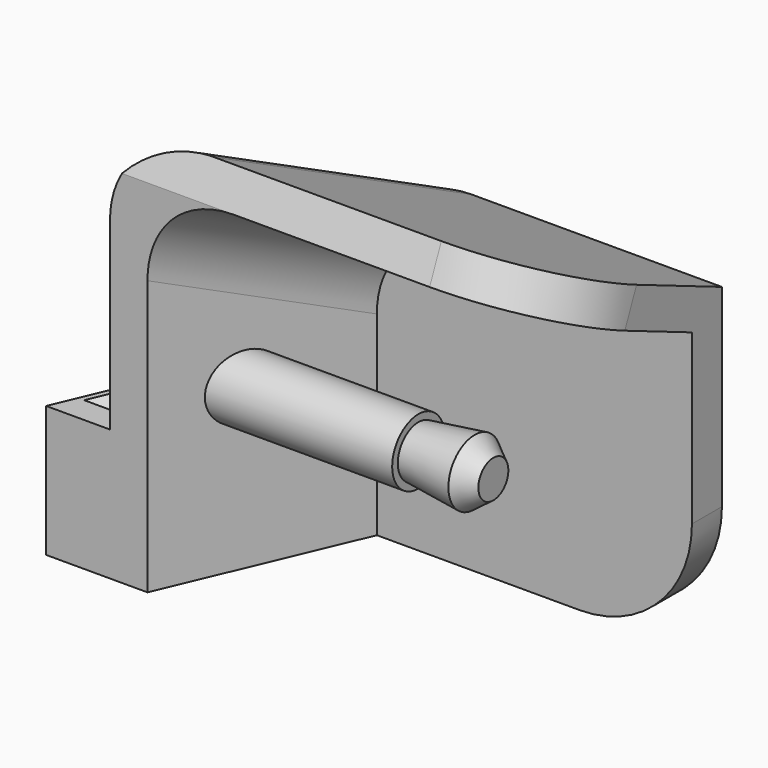
from build123d import *

# Parameters (mm, degrees)
F4_DEPTH      = 20
F4_DEPTH_BACK = 5
F6_DEPTH      = 2
F8_DEPTH      = 2
F10_DEPTH     = 25
F11_REACH     = 32.8764516567
F14_REACH     = 25.371169227
F16_DEPTH     = 7
F17_SIZE      = 1
F18_T4_DEPTH  = 33.0979417074
F18_T8_DEPTH  = 34.519175586


# Not quite as in the source:
# - a fillet or chamfer that OpenCascade refuses, or shapes differently, is made with other operations: its cross-section is extruded or revolved along the edge and cut away or added
# - a feature names something its author has since deleted; it is built from what else it names


with BuildPart() as f1:
    # F0 (on Front) → F1 (revolve)
    with BuildSketch(Plane.XZ):
        Polygon((-4, 1.75), (-14, 1.75), (-14, 0), (0, 0), (0, 1), (-1, 1.75), (-4, 1.375), align=None)
    revolve(axis=Axis((-7, 0, 0), (-1, 0, 0)))


with BuildPart() as f4:
    # F3 (on offset) → F4 (new body, two sides)
    with BuildSketch(Plane(origin=(-14, 0, 0), x_dir=(0, -1, 0), z_dir=(-1, 0, 0))) as f4_sk:
        Polygon((-5.75, 6.5052518379), (4.25, 10.75), (3.468537743, 12.5910097069), (-7.75, 7.8290229603), (-7.75, -8.4947481621), (-5.75, -8.4947481621), align=None)
    extrude(amount=-F4_DEPTH)
    extrude(f4_sk.sketch, amount=F4_DEPTH_BACK)

    # F5 (on face) → F6 (cut, through all)
    with BuildSketch(Plane(origin=(0, 7.75, 0), x_dir=(-1, 0, 0), z_dir=(0, 1, 0))):
        with BuildLine():
            ThreePointArc((0, -8.4947481621), (-4.2426406871, -6.7373888492), (-6, -2.4947481621))
            Line((-6, -2.4947481621), (-6, -8.4947481621))
            Line((-6, -8.4947481621), (0, -8.4947481621))
        make_face()
    extrude(amount=-F6_DEPTH, mode=Mode.SUBTRACT)

    # F7 (on face) → F8 (cut, through all)
    with BuildSketch(Plane(origin=(0, 3.999062721, 9.4212013724), x_dir=(1, 0, 0), z_dir=(0, 0.3907311285, 0.9205048535))):
        with BuildLine():
            ThreePointArc((6, -2.1125052584), (4.2426406871, -6.3551459456), (0, -8.1125052584))
            Line((0, -8.1125052584), (6, -8.1125052584))
            Line((6, -8.1125052584), (6, -2.1125052584))
        make_face()
    extrude(amount=-F8_DEPTH, mode=Mode.SUBTRACT)

    # F9 (on face) → F10 (cut)
    with BuildSketch(Plane(origin=(0, 0, -8.4947481621), x_dir=(1, 0, 0), z_dir=(0, 0, -1))):
        Polygon((-19, -5.75), (-12.8164388784, -5.75), (-17.0611870405, 4.25), (-19, 4.25), align=None)
        Polygon((-19, -7.75), (-11.967489246, -7.75), (-12.8164388784, -5.75), (-19, -5.75), align=None)
    extrude(amount=-F10_DEPTH, mode=Mode.SUBTRACT)

    f11_end = Plane(origin=(-4.5062197261, 2.0556087421, 10.2461486429), x_dir=(0, 0.9205048535, -0.3907311285), z_dir=(0, 0.3907311285, 0.9205048535))
    # F9 (on face) → F11 (join, up to a plane its end follows)
    with BuildSketch(Plane(origin=(0, 0, -8.4947481621), x_dir=(1, 0, 0), z_dir=(0, 0, -1))):
        Polygon((-11.967489246, -7.75), (-9.967489246, -7.75), (-10.8164388784, -5.75), (-12.8164388784, -5.75), align=None)
        Polygon((-12.8164388784, -5.75), (-10.8164388784, -5.75), (-15.0611870405, 4.25), (-17.0611870405, 4.25), align=None)
    f11_long = extrude(amount=-F11_REACH, mode=Mode.PRIVATE)
    add(split(f11_long, bisect_by=f11_end, keep=Keep.BOTTOM, mode=Mode.PRIVATE))

    f14_end = f4.faces().sort_by_distance((-14.6289155357, 1.480072579, 0.9978505439))[0]
    # F13 (on face) → F14 (cut, up to a face of the model that its end follows)
    with BuildSketch(Plane.YZ.offset(6)):
        Polygon((-4.25, 10.75), (-3.468537743, 12.5910097069), (-4.25, 12.9227207548), align=None)
    f14_long = extrude(amount=-F14_REACH, mode=Mode.PRIVATE)
    add(split(f14_long, bisect_by=f14_end, keep=Keep.BOTTOM, mode=Mode.PRIVATE), mode=Mode.SUBTRACT)

    # F15 (on face) → F16 (join)
    with BuildSketch(Plane(origin=(0, 0, -8.4947481621), x_dir=(1, 0, 0), z_dir=(0, 0, -1))):
        with BuildLine():
            Line((-15.3797577366, -7.75), (-11.967489246, -7.75))
            Line((-11.967489246, -7.75), (-12.5606825008, -6.3525242673))
            Line((-12.5606825008, -6.3525242673), (-14.5606825008, -6.3525242673))
            Line((-14.5606825008, -6.3525242673), (-18.4679937857, 2.8525242673))
            Line((-18.4679937857, 2.8525242673), (-16.4679937857, 2.8525242673))
            Line((-16.4679937857, 2.8525242673), (-17.0611870405, 4.25))
            Line((-17.0611870405, 4.25), (-20.4734555312, 4.25))
            Line((-20.4734555312, 4.25), (-17.7109944528, -2.257950467))
            ThreePointArc((-17.7109944528, -2.257950467), (-17.4057692366, -5.1676369709), (-18.7808471141, -7.75))
            Line((-18.7808471141, -7.75), (-15.3797577366, -7.75))
        make_face()
    extrude(amount=-F16_DEPTH)

    # F17
    f17_edges = [f4.edges().sort_by_distance(p)[0] for p in [
        (-16.514338, 1.75, -1.494748),
        (-16.514338, 1.75, -8.494748),
    ]]
    chamfer(f17_edges, length=F17_SIZE)

    # F18: fillet of radius 5 on 2 edges, made by hand


with BuildPart() as f18_tool2:
    # F18_s3 → F18_t4 (new body)
    with BuildSketch(Plane(origin=(3.4003281709, 8.010671166, -3.4003281709), x_dir=(0.9205048535, -0.3907311285, 0), z_dir=(-0.3639362896, -0.857380169, 0.3639362896))):
        with BuildLine():
            ThreePointArc((-12.2032884735, 2.1604142833), (-10.99912635, 5.4148904033), (-7.9666425473, 7.101799773))
            Line((-7.9666425473, 7.101799773), (-12.2032884735, 6.4473151282))
            Line((-12.2032884735, 6.4473151282), (-12.2032884735, 2.1604142833))
        make_face()
    extrude(amount=F18_T4_DEPTH)

    split(bisect_by=Plane.XZ.offset(-5.75), keep=Keep.TOP)

    split(bisect_by=Plane.XZ.offset(4.25), keep=Keep.BOTTOM)

    split(bisect_by=Plane(origin=(0, -7.467600464, 3.1698083345), x_dir=(1, 0, 0), z_dir=(0, 0.9205048535, -0.3907311285)), keep=Keep.TOP)


with BuildPart() as f4_1:
    add(f4.part)

    # F18_t1: union F18_tool2
    add(f18_tool2.part)

    # F18_s9 → F18_t8 (cut)
    with BuildSketch(Plane(origin=(-8.8661781717, -20.8874068216, 8.8661781717), x_dir=(-0.9205048535, 0.3907311285, 0), z_dir=(0.3639362896, 0.857380169, -0.3639362896))):
        with BuildLine():
            ThreePointArc((9.8076522542, 8.841121216), (12.8401360569, 7.1542118462), (14.0442981804, 3.8997357263))
            Line((14.0442981804, 3.8997357263), (14.0442981804, 8.1866365712))
            Line((14.0442981804, 8.1866365712), (9.8076522542, 8.841121216))
        make_face()
    extrude(amount=F18_T8_DEPTH, mode=Mode.SUBTRACT)


solid = Compound([f1.part, f4_1.part])
